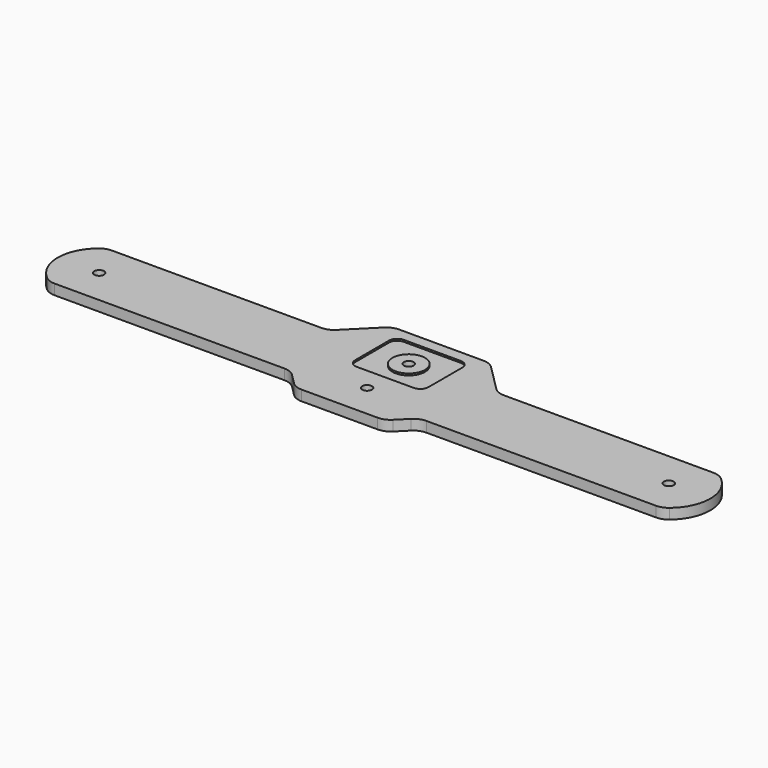
from build123d import *

# Parameters (mm, degrees)
F0_R     = 3
F1_DEPTH = 6.35
F2_R     = 10
F3_R     = 10.5
F4_DEPTH = 2.75
F5_R     = 10
F6_DEPTH = 1.1


# Not quite as in the source:
# - a feature names something its author has since deleted; it is built from what else it names


with BuildPart() as f1:
    # F0 (on Top) → F1 (new body)
    with BuildSketch(Plane.XY):
        with BuildLine():
            Line((25.8578643763, 44), (0, 44))
            Line((0, 44), (-25.8578643763, 44))
            ThreePointArc((-25.8578643763, 44), (-29.6846986999, 43.2387953251), (-32.9289321881, 41.0710678119))
            Line((-32.9289321881, 41.0710678119), (-49.0710678119, 24.9289321881))
            ThreePointArc((-49.0710678119, 24.9289321881), (-52.3153013001, 22.7612046749), (-56.1421356237, 22))
            Line((-56.1421356237, 22), (-187.8528743982, 22))
            ThreePointArc((-187.8528743982, 22), (-200.4793324147, 0), (-187.8528743982, -22))
            Line((-187.8528743982, -22), (-43.6421356237, -22))
            ThreePointArc((-43.6421356237, -22), (-39.8153013001, -22.7612046749), (-36.5710678119, -24.9289321881))
            Line((-36.5710678119, -24.9289321881), (-30.4289321881, -31.0710678119))
            ThreePointArc((-30.4289321881, -31.0710678119), (-27.1846986999, -33.2387953251), (-23.3578643763, -34))
            Line((-23.3578643763, -34), (0, -34))
            Line((0, -34), (23.3578643763, -34))
            ThreePointArc((23.3578643763, -34), (27.1846986999, -33.2387953251), (30.4289321881, -31.0710678119))
            Line((30.4289321881, -31.0710678119), (36.5710678119, -24.9289321881))
            ThreePointArc((36.5710678119, -24.9289321881), (39.8153013001, -22.7612046749), (43.6421356237, -22))
            Line((43.6421356237, -22), (187.8528743982, -22))
            ThreePointArc((187.8528743982, -22), (200.4793324147, 0), (187.8528743982, 22))
            Line((187.8528743982, 22), (56.1421356237, 22))
            ThreePointArc((56.1421356237, 22), (52.3153013001, 22.7612046749), (49.0710678119, 24.9289321881))
            Line((49.0710678119, 24.9289321881), (32.9289321881, 41.0710678119))
            ThreePointArc((32.9289321881, 41.0710678119), (29.6846986999, 43.2387953251), (25.8578643763, 44))
        make_face()
        with Locations((-175, 0)):
            Circle(F0_R, mode=Mode.SUBTRACT)
        with Locations((0, -13)):
            Circle(F0_R, mode=Mode.SUBTRACT)
        with Locations((175, 0)):
            Circle(F0_R, mode=Mode.SUBTRACT)
        with Locations((0, 19)):
            Circle(F0_R, mode=Mode.SUBTRACT)
    extrude(amount=F1_DEPTH)

    # F2
    f2_edges = [f1.edges().sort_by_distance(p)[0] for p in [
        (-187.852874, 22, 3.175),
        (-187.852874, -22, 3.175),
        (187.852874, -22, 3.175),
        (187.852874, 22, 3.175),
    ]]
    fillet(f2_edges, radius=F2_R)

    # F3 (on face) → F4 (cut)
    with BuildSketch(Plane(origin=(0, 0, 0), x_dir=(1, 0, 0), z_dir=(0, 0, -1))):
        with Locations((0, -19)):
            Circle(F3_R)
    extrude(amount=-F4_DEPTH, mode=Mode.SUBTRACT)

    # F5 (on face) → F6 (cut)
    with BuildSketch(Plane.XY.offset(6.35)):
        with BuildLine():
            ThreePointArc((22.5, 32), (21.0355339059, 35.5355339059), (17.5, 37))
            Line((17.5, 37), (-17.5, 37))
            ThreePointArc((-17.5, 37), (-21.0355339059, 35.5355339059), (-22.5, 32))
            Line((-22.5, 32), (-22.5, 6))
            ThreePointArc((-22.5, 6), (-21.0355339059, 2.4644660941), (-17.5, 1))
            Line((-17.5, 1), (17.5, 1))
            ThreePointArc((17.5, 1), (21.0355339059, 2.4644660941), (22.5, 6))
            Line((22.5, 6), (22.5, 32))
        make_face()
        with Locations((0, 19)):
            Circle(F5_R, mode=Mode.SUBTRACT)
    extrude(amount=-F6_DEPTH, mode=Mode.SUBTRACT)


solid = f1.part
